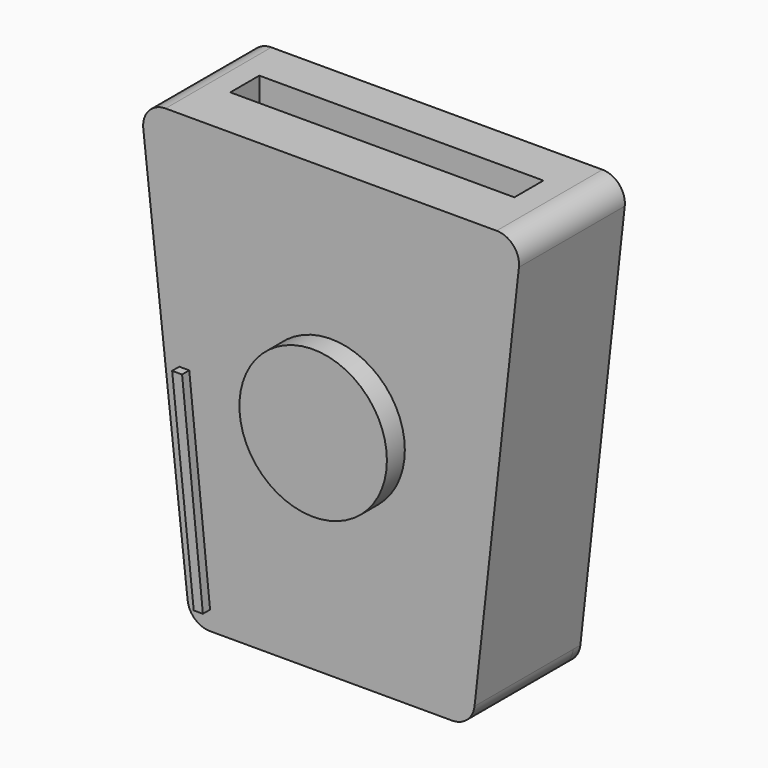
from build123d import *

# Parameters (mm, degrees)
F1_DEPTH   = 6.985
F2_R       = 4.1774350827
F3_DEPTH   = 1.27
F6_DEPTH   = 0.508
F8_DEPTH   = 0.508
F9_R       = 1.27
F10_W      = 16.0917048343
F10_H      = 2.0555099472
F8_FACE1_W = 13.7275979897
F8_FACE1_H = 7.493
F11_DEPTH  = 5.08
F12_W      = 10.965348687
F12_H      = 1.5682033263
F13_DEPTH  = 5.08


# Not quite as in the source:
# - a feature names something its author has since deleted; it is built from what else it names


with BuildPart() as f1:
    # F0 (on Front) → F1 (new body)
    with BuildSketch(Plane.XZ):
        Polygon((10.795, 12.6229311572), (-10.795, 12.6229311572), (-8.001, -12.6229311572), (8.001, -12.6229311572), align=None)
    extrude(amount=-F1_DEPTH)

    # F2 (on face) → F3 (join)
    with BuildSketch(Plane.XZ):
        Circle(F2_R)
    extrude(amount=F3_DEPTH)

    # F5 (on face) + F1_face1 (on face) → F6 (join)
    with BuildSketch(Plane.XZ):
        Polygon((-8.0337325091, 0), (-8.597294162, 0), (-7.3735090208, -11.5506481379), (-6.855092685, -11.5506481379), align=None)
    with BuildSketch(Plane(origin=(0, 6.985, 0.6254605528), x_dir=(1, 0, 0), z_dir=(0, 1, 0))):
        Polygon((-10.795, -11.9974706044), (10.795, -11.9974706044), (8.001, 13.2483917101), (-8.001, 13.2483917101), align=None)
    extrude(amount=F6_DEPTH, dir=(0, -1, 0))

    # F7 (on face) → F8 (join)
    with BuildSketch(Plane(origin=(0, 6.985, 0), x_dir=(-1, 0, 0), z_dir=(0, 1, 0))):
        Polygon((8.001, -12.6229311572), (10.795, 12.6229311572), (-10.795, 12.6229311572), (-8.001, -12.6229311572), align=None)
        Polygon((8.051493348, 0), (8.559493348, 0), (7.418411777, -11.551577974), (6.910411777, -11.551577974), align=None, mode=Mode.SUBTRACT)
    extrude(amount=F8_DEPTH)

    # F9
    f9_edges = [f1.edges().sort_by_distance(p)[0] for p in [
        (-10.795, 3.7465, 12.622931),
        (10.795, 3.7465, 12.622931),
        (8.001, 3.7465, -12.622931),
        (-8.001, 3.7465, -12.622931),
    ]]
    fillet(f9_edges, radius=F9_R)

    # F10 (on face) + F8_face1 (on face) → F11 (cut)
    with BuildSketch(Plane.XY.offset(12.6229311572)):
        with Locations((-0.0573594589, 4.0197446942)):
            Rectangle(F10_W, F10_H)
    with BuildSketch(Plane(origin=(0, 3.7465, -12.6229311572), x_dir=(1, 0, 0), z_dir=(0, 0, -1))):
        Rectangle(F8_FACE1_W, F8_FACE1_H)
    extrude(amount=-F11_DEPTH, dir=(0, 0, 1), mode=Mode.SUBTRACT)

    # F12 (on face) → F13 (cut)
    with BuildSketch(Plane(origin=(0, 0, -12.6229311572), x_dir=(1, 0, 0), z_dir=(0, 0, -1))):
        with Locations((-0.0077148434, -3.7751414347)):
            Rectangle(F12_W, F12_H)
    extrude(amount=-F13_DEPTH, mode=Mode.SUBTRACT)


solid = f1.part
